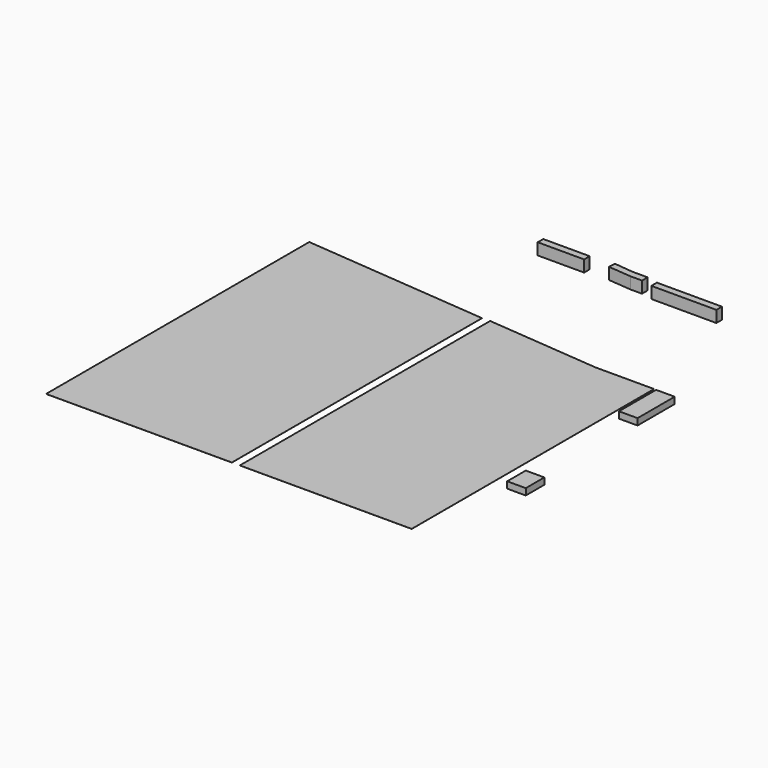
from build123d import *

# Parameters (mm, degrees)
F0_W     = 400
F0_H     = 1000
F1_DEPTH = 140
F0_H_2   = 500
F2_DEPTH = 1
F4_DEPTH = 1
F0_W_2   = 1000
F0_H_3   = 150
F6_DEPTH = 250
F0_W_3   = 1400


# Not quite as in the source:
# - the program builds the solid bodies; features that only make, move or delete a surface that nothing else refers to are left out


with BuildPart() as f1:
    # F0 (on Top) → F1 (new body)
    with BuildSketch(Plane.XY):
        with Locations((3308.4599494934, 4327.3605238324)):
            Rectangle(F0_W, F0_H)
    extrude(amount=-F1_DEPTH)


with BuildPart() as f1b:
    # F0 (on Top) → F1, piece 2 (new body)
    with BuildSketch(Plane.XY):
        with Locations((3432.9387664795, 913.2413864136)):
            Rectangle(F0_W, F0_H_2)
    extrude(amount=-F1_DEPTH)


with BuildPart() as f2:
    # F0 (on Top) → F2 (new body)
    with BuildSketch(Plane.XY):
        Polygon((-4808.1577976546, -1695.3865286843), (-808.1577976546, -1695.3865286843), (-808.1577976546, 5037.3098283165), (-4808.1577976546, 5387.2644824202), align=None)
    extrude(amount=-F2_DEPTH)


with BuildPart() as f4:
    # F0 (on Top) → F4 (new body)
    with BuildSketch(Plane.XY):
        Polygon((-636.1389268665, 5040.8328628357), (-636.1389268665, -1695.3865286843), (3063.8610731335, -1695.3865286843), (3063.8610731335, 4827.3605238324), (1803.8610731335, 4827.3605238324), align=None)
    extrude(amount=F4_DEPTH)


with BuildPart() as f6:
    # F0 (on Top) → F6 (new body)
    with BuildSketch(Plane.XY):
        with Locations((-1002.815246582, 7479.6626091003)):
            Rectangle(F0_W_2, F0_H_3)
    extrude(amount=F6_DEPTH)


with BuildPart() as f6b:
    # F0 (on Top) → F6, piece 2 (new body)
    with BuildSketch(Plane.XY):
        Polygon((487.73180431, 7411.6362518106), (737.73180431, 7411.6362518106), (737.73180431, 7561.6362518106), (417.8309041372, 7561.6362518106), (2.7078166763, 7604.6433278982), (-10.3655447358, 7455.2141231845), align=None)
    extrude(amount=F6_DEPTH)


with BuildPart() as f6c:
    # F0 (on Top) → F6, piece 3 (new body)
    with BuildSketch(Plane.XY):
        with Locations((1679.790687561, 7434.1046333313)):
            Rectangle(F0_W_3, F0_H_3)
    extrude(amount=F6_DEPTH)


solid = Compound([f1.part, f1b.part, f2.part, f4.part, f6.part, f6b.part, f6c.part])
